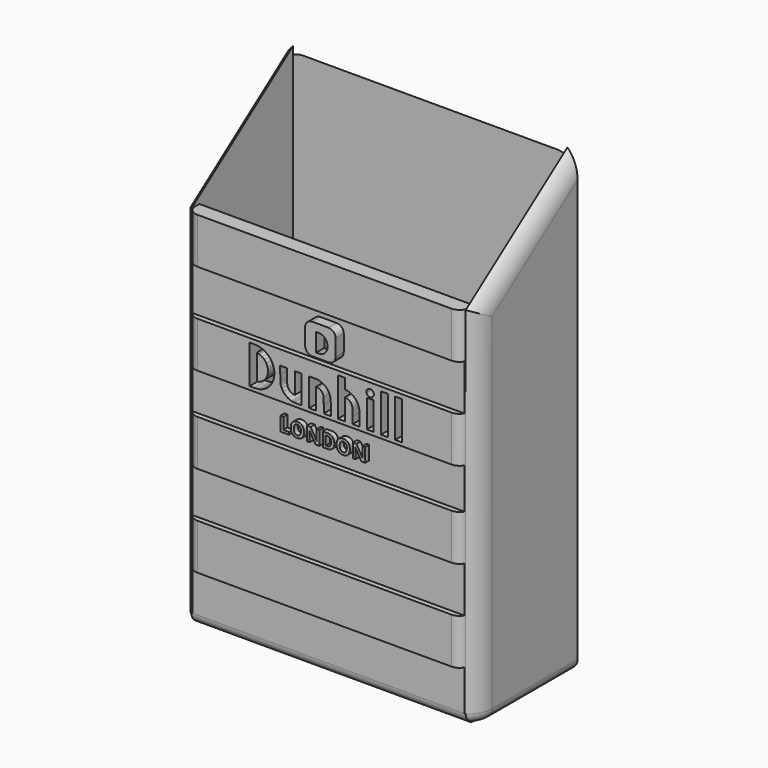
from build123d import *

# Parameters (mm, degrees)
F0_W           = 54
F0_H           = 25
F2_DEPTH       = 2
F9_DEPTH       = 2
F4_W           = 54
F4_H           = 70
F10_DEPTH      = 2
F11_DEPTH      = 2
F1_W           = 58
F1_H           = 90
F12_DEPTH      = 2
F13_T1_DEPTH   = 92
F13_2_T1_DEPTH = 92
F13_3_T1_DEPTH = 110
F14_R          = 1.99999
F14_2_R        = 1.99999
F14_3_R        = 1.99999
F15_R          = 1.99999
F16_W          = 54
F16_H          = 9
F17_DEPTH      = 1
F18_F1_R       = 2
F18_F2_R       = 1.9996
F20_DEPTH      = 3
F21_TEXT_SIZE  = 3.8399082091
F22_DEPTH      = 1
F23_W          = 6
F23_H          = 6
F24_DEPTH      = 2
F25_R          = 1.4
F27_DEPTH      = 2
F28_T1_DEPTH   = 45.8860060935
F28_2_T1_DEPTH = 45.8389282305
F28_3_T1_DEPTH = 50
F28_3_T4_ANGLE = 196.3896000127
F28_3_T6_ANGLE = 196.3896000127


# Not quite as in the source:
# - a fillet or chamfer that OpenCascade refuses, or shapes differently, is made with other operations: its cross-section is extruded or revolved along the edge and cut away or added
# - a fillet or chamfer is up to 0.001 mm smaller than in the source, because OpenCascade refuses the exact size
# - Text() gives the source's letters only with a copy of the font that has no kerning and outlines rounded to 1/6400 em; it was checked with that copy


with BuildPart() as f2:
    # F0 (on Top) → F2 (new body)
    with BuildSketch(Plane.XY):
        with Locations((23.2370707691, -12.5)):
            Rectangle(F0_W, F0_H)
    extrude(amount=-F2_DEPTH)

    # F15 (radius 2 in the source; OpenCascade refuses exactly that, so slightly less here)
    f15_edges = [f2.edges().sort_by_distance(p)[0] for p in [
        (23.237071, -25, -2),
    ]]
    fillet(f15_edges, radius=F15_R)


with BuildPart() as f9:
    # F6 (on offset) → F9 (new body)
    with BuildSketch(Plane.YZ.offset(50.2370707691)):
        Polygon((-25, 70), (-25, -2), (0, -2), (0, 88.0185291171), align=None)
    extrude(amount=F9_DEPTH)

    # F13: fillet of radius 5 on 1 edges, made by hand

    # F13_s2 → F13_t1 (cut)
    with BuildSketch(Plane.XY.offset(-12)):
        with BuildLine():
            ThreePointArc((50.2370707691, -25), (51.7092067241, -23.2360679775), (52.2370707691, -21))
            Line((52.2370707691, -21), (52.2370707691, -25))
            Line((52.2370707691, -25), (50.2370707691, -25))
        make_face()
    extrude(amount=F13_T1_DEPTH, mode=Mode.SUBTRACT)

    # F14 (radius 2 in the source; OpenCascade refuses exactly that, so slightly less here)
    f14_edges = [f9.edges().sort_by_distance(p)[0] for p in [
        (52.237071, -10.5, -2),
    ]]
    fillet(f14_edges, radius=F14_R)

    # F28: fillet of radius 5 on 1 edges, made by hand

    # F28_s2 → F28_t1 (cut)
    with BuildSketch(Plane(origin=(0, 49.8630148254, 35.9383273799), x_dir=(1, 0, 0), z_dir=(0, -0.811249133, -0.584700645))):
        with BuildLine():
            ThreePointArc((50.2370707691, 71.4049554335), (51.7092067241, 69.641023411), (52.2370707691, 67.4049554335))
            Line((52.2370707691, 67.4049554335), (52.2370707691, 71.4049554335))
            Line((52.2370707691, 71.4049554335), (50.2370707691, 71.4049554335))
        make_face()
    extrude(amount=F28_T1_DEPTH, mode=Mode.SUBTRACT)


with BuildPart() as f10:
    # F4 (on offset) → F10 (new body)
    with BuildSketch(Plane.XZ.offset(23)):
        with Locations((23.2337976322, 35)):
            Rectangle(F4_W, F4_H)
    extrude(amount=F10_DEPTH)

    # F16 (on face) → F17 (join)
    with BuildSketch(Plane.XZ.offset(25)):
        with Locations((23.2337976322, 65.5)):
            Rectangle(F16_W, F16_H)
        with Locations((23.2337976322, 47.5)):
            Rectangle(F16_W, F16_H)
        with Locations((23.2337976322, 30.5)):
            Rectangle(F16_W, F16_H)
        with Locations((23.2337976322, 12.5)):
            Rectangle(F16_W, F16_H)
    extrude(amount=F17_DEPTH)

    # F18: fillet of radius 2 on 8 edges, made by hand

    # F18_f1
    f18_f1_edges = [f10.edges().sort_by_distance(p)[0] for p in [
        (-3.7662023678, -26, 47.5),
    ]]
    fillet(f18_f1_edges, radius=F18_F1_R)

    # F18_f2 (radius 2 in the source; OpenCascade refuses exactly that, so slightly less here)
    f18_f2_edges = [f10.edges().sort_by_distance(p)[0] for p in [
        (50.2337976322, -26, 12.5),
    ]]
    fillet(f18_f2_edges, radius=F18_F2_R)

    # F19 (on face) → F20 (cut)
    with BuildSketch(Plane.XZ.offset(26)):
        with BuildLine():
            Line((8.4967808397, 51.220968125), (8.4967808397, 47.4348578924))
            Line((8.4967808397, 47.4348578924), (8.4967808397, 43.6487476599))
            Line((8.4967808397, 43.6487476599), (9.368873863, 43.668248809))
            ThreePointArc((9.3688738631, 43.6682488024), (9.7077723614, 43.6793255754), (10.0463702246, 43.6973914009))
            ThreePointArc((10.0463702223, 43.6973914371), (10.266896193, 43.7191683277), (10.4853730632, 43.7562330531))
            ThreePointArc((10.4853730706, 43.7562330175), (10.6760414895, 43.8040619553), (10.8619078322, 43.8680600487))
            ThreePointArc((10.8619078192, 43.8680600818), (11.0872012313, 43.9625459733), (11.3079983364, 44.0671086035))
            ThreePointArc((11.3079983468, 44.0671085827), (11.6452174269, 44.2584053812), (11.9611395896, 44.483137133))
            ThreePointArc((11.9611395912, 44.483137131), (12.2508833738, 44.7379466338), (12.5126747359, 45.0213979082))
            ThreePointArc((12.5126747117, 45.0213979284), (12.7444666513, 45.3313556173), (12.943023476, 45.6635851457))
            ThreePointArc((12.9430235242, 45.6635851201), (13.1084809679, 46.0179285104), (13.2376405598, 46.3870534266))
            ThreePointArc((13.2376405484, 46.3870534299), (13.2909037655, 46.5945265675), (13.3294551184, 46.8052298334))
            ThreePointArc((13.3294551154, 46.8052298339), (13.3574144288, 47.0387027013), (13.3729137893, 47.2733323517))
            ThreePointArc((13.3729137735, 47.2733323524), (13.3759300416, 47.509092507), (13.3664249519, 47.744680286))
            ThreePointArc((13.36642497, 47.7446802873), (13.3445612976, 47.9596933996), (13.3079449581, 48.1726908229))
            ThreePointArc((13.3079449225, 48.1726908155), (13.1932583708, 48.6006717625), (13.0305332816, 49.0127897571))
            ThreePointArc((13.0305333058, 49.0127897683), (12.82358236, 49.3985536561), (12.5725005259, 49.7571626126))
            ThreePointArc((12.5725005308, 49.7571626165), (12.2803608082, 50.084163496), (11.9516949748, 50.3744288275))
            ThreePointArc((11.9516949682, 50.374428819), (11.5863213494, 50.6286025823), (11.1946065561, 50.8399357408))
            ThreePointArc((11.1946065575, 50.8399357437), (10.9931829534, 50.9280602816), (10.787480949, 51.005675279))
            ThreePointArc((10.7874809466, 51.0056752723), (10.6003517758, 51.0632567232), (10.4095232186, 51.1070449848))
            ThreePointArc((10.4095232219, 51.107045002), (10.1878049733, 51.1427450964), (9.9643702521, 51.1653372164))
            ThreePointArc((9.9643702512, 51.1653372049), (9.6462722249, 51.1846554218), (9.3278341912, 51.1971760702))
            Line((9.3278341913, 51.197176073), (8.4967808397, 51.220968125))
        make_face()
        with BuildLine():
            ThreePointArc((10.3421098572, 49.8377194327), (10.3942364029, 49.821717243), (10.4461652473, 49.8050846858))
            ThreePointArc((10.4461652344, 49.8050846463), (10.7123895905, 49.6984875575), (10.9625976621, 49.5583652251))
            ThreePointArc((10.9625976924, 49.5583652719), (11.2036710915, 49.3816313865), (11.4229646443, 49.1785019016))
            ThreePointArc((11.4229646233, 49.1785018814), (11.6208645225, 48.9482688721), (11.7916159508, 48.6972398729))
            ThreePointArc((11.79161596, 48.6972398784), (11.930667684, 48.4317134841), (12.0377438832, 48.1517593172))
            ThreePointArc((12.037743906, 48.1517593244), (12.0838629347, 47.9778393221), (12.113258297, 47.8003258165))
            ThreePointArc((12.1132582866, 47.8003258153), (12.1300120701, 47.5988487204), (12.1332024594, 47.3967014215))
            ThreePointArc((12.1332024459, 47.3967014217), (12.1227781224, 47.1934925842), (12.0987956049, 46.9914348274))
            ThreePointArc((12.0987955999, 46.9914348282), (12.0628385981, 46.8111503169), (12.0107246706, 46.6348563875))
            ThreePointArc((12.0107246527, 46.6348563937), (11.8929420091, 46.3494845152), (11.7425269104, 46.0798826638))
            ThreePointArc((11.7425269194, 46.0798826581), (11.5620601339, 45.8308124438), (11.3533507512, 45.6048818663))
            ThreePointArc((11.3533507478, 45.6048818699), (11.1202369481, 45.4061489653), (10.8651243479, 45.2365778234))
            ThreePointArc((10.8651243526, 45.2365778153), (10.5925010557, 45.0992258668), (10.3053375694, 44.9956587298))
            ThreePointArc((10.3053375696, 44.9956587292), (10.1899858789, 44.9766548845), (10.0734708548, 44.986215628))
            ThreePointArc((10.0734708495, 44.9862156028), (10.0002728859, 45.0269816707), (9.9634339656, 45.1022326383))
            ThreePointArc((9.9634339712, 45.1022326392), (9.9428673797, 45.2813766604), (9.9356912782, 45.4615545409))
            ThreePointArc((9.9356912776, 45.4615545409), (9.9337995981, 46.4470459979), (9.9331693487, 47.4325390689))
            Line((9.9331693486, 47.4325390689), (9.9331693486, 49.9349330497))
            Line((9.9331693486, 49.9349330497), (10.0665482816, 49.91026714))
            ThreePointArc((10.066548282, 49.910267142), (10.10056304, 49.9033961224), (10.1343333028, 49.8954096324))
            ThreePointArc((10.1343333037, 49.895409636), (10.1837772482, 49.8825691283), (10.2330795556, 49.8691950946))
            ThreePointArc((10.233079556, 49.8691950959), (10.2876793131, 49.8537503375), (10.3421098571, 49.8377194322))
        make_face(mode=Mode.SUBTRACT)
        with BuildLine():
            Line((25.8976016332, 51.2092148555), (25.8976016332, 47.4335650607))
            Line((25.8976016332, 47.4335650607), (25.8976016332, 43.6579152659))
            Line((25.8976016332, 43.6579152659), (26.5747562159, 43.6579152659))
            Line((26.5747562159, 43.6579152659), (27.2519107987, 43.6579152659))
            Line((27.2519107987, 43.6579152659), (27.2519107987, 45.7361351428))
            Line((27.2519107987, 45.7361351428), (27.2519107987, 47.8143550196))
            Line((27.2519107987, 47.8143550196), (27.4602764348, 47.7896771674))
            ThreePointArc((27.4602764366, 47.7896771826), (27.6229020401, 47.7600920806), (27.7806130739, 47.7105986973))
            ThreePointArc((27.7806130713, 47.7105986903), (27.9373517472, 47.6403229619), (28.085370267, 47.5531667323))
            ThreePointArc((28.085370265, 47.5531667294), (28.2217245815, 47.4509514822), (28.3458536199, 47.3341934495))
            ThreePointArc((28.3458536112, 47.3341934412), (28.4492623182, 47.2101111114), (28.5355912966, 47.0735933736))
            ThreePointArc((28.5355913081, 47.0735933798), (28.6076371898, 46.9252978609), (28.6656963831, 46.7709887552))
            ThreePointArc((28.6656963911, 46.7709887578), (28.7075850332, 46.6158854669), (28.7338101803, 46.4573801645))
            ThreePointArc((28.7338101596, 46.4573801622), (28.7545565402, 46.2249601835), (28.763644156, 45.9917931317))
            ThreePointArc((28.7636441641, 45.9917931318), (28.7686951555, 45.5079692206), (28.7703786509, 45.0241218733))
            Line((28.770378651, 45.0241218733), (28.770378651, 43.6579152659))
            Line((28.770378651, 43.6579152659), (29.4475332337, 43.6579152659))
            Line((29.4475332337, 43.6579152659), (30.1246878165, 43.6579152659))
            Line((30.1246878165, 43.6579152659), (30.1243778028, 45.0224843493))
            ThreePointArc((30.1243778036, 45.0224843493), (30.1235330819, 45.2944295527), (30.1211230705, 45.566365389))
            ThreePointArc((30.1211230767, 45.5663653891), (30.1172633689, 45.8160885378), (30.1115488496, 46.0657761279))
            ThreePointArc((30.1115488419, 46.0657761277), (30.1053866555, 46.2743546576), (30.0979989786, 46.482893378))
            ThreePointArc((30.0979990012, 46.4828933789), (30.0920925158, 46.5686115086), (30.0809803833, 46.6538113023))
            ThreePointArc((30.0809803539, 46.6538112976), (29.9992595289, 47.0168027816), (29.8737606722, 47.3670757432))
            ThreePointArc((29.8737606904, 47.3670757511), (29.7073423227, 47.6960324996), (29.5008948305, 48.0014617852))
            ThreePointArc((29.5008948152, 48.0014617734), (29.2565085481, 48.2800852993), (28.9792278131, 48.525994044))
            ThreePointArc((28.9792278008, 48.5259940283), (28.6684591584, 48.7402404835), (28.3345250977, 48.9162141628))
            ThreePointArc((28.3345251138, 48.9162141984), (28.2184154982, 48.9656102913), (28.1001164396, 49.0095050471))
            ThreePointArc((28.100116427, 49.0095050105), (27.9726735504, 49.0506384212), (27.8437141442, 49.0867371167))
            ThreePointArc((27.8437141557, 49.0867371612), (27.7221838754, 49.1155868542), (27.5995860553, 49.1394968592))
            ThreePointArc((27.5995860522, 49.1394968417), (27.5030586417, 49.1521430432), (27.4058095675, 49.1566246663))
            Line((27.4058095675, 49.156624664), (27.2519107987, 49.1572312714))
            Line((27.2519107987, 49.1572312714), (27.2519107987, 50.1832230634))
            Line((27.2519107987, 50.1832230634), (27.2519107987, 51.2092148555))
            Line((27.2519107987, 51.2092148555), (26.5747562159, 51.2092148555))
            Line((26.5747562159, 51.2092148555), (25.8976016332, 51.2092148555))
        make_face()
        Polygon((34.3517739998, 51.1681751838), (34.3517739998, 47.4130452248), (34.3517739998, 43.6579152659), (35.0289285826, 43.6579152659), (35.7060831653, 43.6579152659), (35.7060831653, 47.4130452248), (35.7060831653, 51.1681751838), (35.0289285826, 51.1681751838), align=None)
        Polygon((37.1424716742, 51.1681751838), (37.1424716742, 47.4130452248), (37.1424716742, 43.6579152659), (37.819626257, 43.6579152659), (38.4967808397, 43.6579152659), (38.4967808397, 47.4130452248), (38.4967808397, 51.1681751838), (37.819626257, 51.1681751838), align=None)
        with BuildLine():
            ThreePointArc((32.1791323452, 50.8734274335), (32.0340379968, 50.8460404102), (31.896299571, 50.7928375433))
            ThreePointArc((31.8962995589, 50.7928375677), (31.7524013071, 50.6990758408), (31.6343795702, 50.5743006913))
            ThreePointArc((31.634379585, 50.5743006803), (31.5502098515, 50.4266613576), (31.5040648836, 50.2630992728))
            ThreePointArc((31.5040648713, 50.2630992747), (31.4984281146, 50.0921051918), (31.533746399, 49.9247033752))
            ThreePointArc((31.5337463815, 49.9247033692), (31.608345886, 49.7673183857), (31.7166586456, 49.6309238652))
            ThreePointArc((31.7166586768, 49.6309238964), (31.8507479036, 49.5245760291), (32.0055320329, 49.4515577919))
            ThreePointArc((32.0055320209, 49.4515577564), (32.1702777175, 49.4172739814), (32.3384419099, 49.4233834952))
            ThreePointArc((32.3384419082, 49.4233835056), (32.5000557816, 49.4695088239), (32.6459142045, 49.553006785))
            ThreePointArc((32.6459142072, 49.5530067814), (32.7700648801, 49.6701605911), (32.8640859039, 49.8126332263))
            ThreePointArc((32.8640859055, 49.8126332255), (32.9003694958, 49.8944319986), (32.9282558218, 49.9794607645))
            ThreePointArc((32.9282558337, 49.9794607613), (32.9453784748, 50.0615673922), (32.9523778003, 50.1451478511))
            ThreePointArc((32.9523778003, 50.1451478511), (32.9490635085, 50.2265235807), (32.9355120586, 50.3068314391))
            ThreePointArc((32.9355120386, 50.3068314344), (32.9117988891, 50.3860704491), (32.8787128437, 50.4618757822))
            ThreePointArc((32.8787128446, 50.4618757826), (32.7993813787, 50.5881573548), (32.6989463261, 50.6983994391))
            ThreePointArc((32.6989463218, 50.6983994344), (32.5855016264, 50.7825875652), (32.4570587006, 50.8414072481))
            ThreePointArc((32.4570587041, 50.8414072585), (32.319784733, 50.8720792133), (32.179132345, 50.8734274359))
        make_face()
        with BuildLine():
            Line((14.5241674334, 49.1572312714), (14.5396058192, 47.649023337))
            ThreePointArc((14.5396058039, 47.6490233369), (14.5467193462, 47.1057908162), (14.5569389503, 46.5626078511))
            ThreePointArc((14.5569389723, 46.5626078515), (14.5682483481, 46.3277414503), (14.5919581248, 46.0938013407))
            ThreePointArc((14.591958115, 46.0938013394), (14.6227813362, 45.9232944126), (14.6709369932, 45.7568500803))
            ThreePointArc((14.6709369781, 45.7568500751), (14.7464050066, 45.5567226203), (14.8327948173, 45.3610616327))
            ThreePointArc((14.8327948066, 45.3610616276), (14.9765414947, 45.0939940481), (15.1464320066, 44.8427463291))
            ThreePointArc((15.1464320149, 44.8427463353), (15.3378461137, 44.6146663753), (15.5524214036, 44.4082268678))
            ThreePointArc((15.5524214239, 44.4082268912), (15.7931668258, 44.2209742962), (16.0519744034, 44.0596035411))
            ThreePointArc((16.0519743908, 44.0596035182), (16.3418650995, 43.9150619759), (16.6431556653, 43.7960961178))
            ThreePointArc((16.643155674, 43.796096143), (16.7521732863, 43.7610037313), (16.862592786, 43.7306088099))
            ThreePointArc((16.8625927853, 43.7306088074), (16.95719232, 43.7102578507), (17.0529921133, 43.6966331311))
            ThreePointArc((17.052992113, 43.6966331283), (17.182524932, 43.6853873594), (17.3123959973, 43.679164428))
            ThreePointArc((17.3123959963, 43.6791643911), (17.5882244819, 43.6719989595), (17.8640859008, 43.6662392338))
            Line((17.8640859013, 43.6662392604), (18.7566987604, 43.6498773999))
            Line((18.7566987604, 43.6498773999), (18.7566987604, 46.4035543357))
            Line((18.7566987604, 46.4035543357), (18.7566987604, 49.1572312714))
            Line((18.7566987604, 49.1572312714), (18.0795441776, 49.1572312714))
            Line((18.0795441776, 49.1572312714), (17.4023895949, 49.1572312714))
            Line((17.4023895949, 49.1572312714), (17.4023895949, 47.0811205463))
            Line((17.4023895949, 47.0811205463), (17.4023895949, 45.0050098213))
            Line((17.4023895949, 45.0050098213), (17.2279709902, 45.0340384943))
            ThreePointArc((17.22797099, 45.0340384932), (17.1864201049, 45.0417336558), (17.1451768588, 45.0509361683))
            ThreePointArc((17.145176862, 45.0509361814), (17.091714273, 45.0643642451), (17.038483114, 45.0786822413))
            ThreePointArc((17.0384831181, 45.0786822558), (16.9826073956, 45.0947100997), (16.9270036524, 45.1116574263))
            ThreePointArc((16.9270036391, 45.1116573839), (16.8772295139, 45.1278964082), (16.8278341858, 45.145253568))
            ThreePointArc((16.8278341929, 45.1452535875), (16.705645414, 45.1996183167), (16.5921582152, 45.2703733671))
            ThreePointArc((16.5921582341, 45.2703733932), (16.4667498542, 45.3693126192), (16.3498733129, 45.478198368))
            ThreePointArc((16.3498733067, 45.4781983619), (16.2401345989, 45.5985830867), (16.1405164838, 45.7274679078))
            ThreePointArc((16.1405164615, 45.7274678919), (16.0646729637, 45.8489941712), (16.0037899213, 45.9786634731))
            ThreePointArc((16.0037899231, 45.9786634738), (15.9709237931, 46.0730990143), (15.9465946961, 46.1700853477))
            ThreePointArc((15.9465946649, 46.1700853413), (15.9283888077, 46.277981146), (15.9175671406, 46.3868657152))
            ThreePointArc((15.917567196, 46.3868657188), (15.9081505372, 46.5671045351), (15.9033557332, 46.7475254714))
            ThreePointArc((15.9033556986, 46.7475254709), (15.8973680354, 47.2187884673), (15.8923709791, 47.6900630086))
            Line((15.8923709902, 47.6900630087), (15.8783553678, 49.1572312714))
            Line((15.8783553678, 49.1572312714), (15.2012614006, 49.1572312714))
            Line((15.2012614006, 49.1572312714), (14.5241674334, 49.1572312714))
        make_face()
        with BuildLine():
            Line((20.234126941, 49.1572312714), (20.234126941, 46.4075732686))
            Line((20.234126941, 46.4075732686), (20.234126941, 43.6579152659))
            Line((20.234126941, 43.6579152659), (20.9112815237, 43.6579152659))
            Line((20.9112815237, 43.6579152659), (21.5884361065, 43.6579152659))
            Line((21.5884361065, 43.6579152659), (21.5884361065, 45.7304186859))
            Line((21.5884361065, 45.7304186859), (21.5884361065, 47.8029221058))
            Line((21.5884361065, 47.8029221058), (21.7072322077, 47.8029221058))
            ThreePointArc((21.7072322077, 47.8029221058), (21.7388715452, 47.8015985367), (21.7702897864, 47.7976370168))
            ThreePointArc((21.7702897858, 47.7976370136), (21.8202969528, 47.7886311323), (21.8700950251, 47.7785328826))
            ThreePointArc((21.8700950252, 47.7785328831), (21.9268009471, 47.7657297455), (21.9832103329, 47.7516775887))
            ThreePointArc((21.9832103366, 47.7516776032), (22.0392009393, 47.7364057299), (22.0948388186, 47.7198950037))
            ThreePointArc((22.0948388063, 47.7198949639), (22.2266138218, 47.670790851), (22.3519319459, 47.6069846099))
            ThreePointArc((22.3519319597, 47.6069846335), (22.4741158004, 47.5270829932), (22.5875148594, 47.4351383551))
            ThreePointArc((22.5875148652, 47.4351383615), (22.6946268006, 47.3288223536), (22.7907531671, 47.2124789745))
            ThreePointArc((22.790753173, 47.2124789789), (22.8774322212, 47.0845045132), (22.9520156122, 46.9491234249))
            Line((22.9520156003, 46.9491234191), (23.0863841229, 46.6763073179))
            Line((23.0863841229, 46.6763073179), (23.0985330969, 45.1671112714))
            Line((23.0985330969, 45.1671112714), (23.1106820709, 43.6579152659))
            Line((23.1106820709, 43.6579152659), (23.8107081448, 43.6579152659))
            Line((23.8107081448, 43.6579152659), (24.5107342187, 43.6579152659))
            Line((24.5107342187, 43.6579152659), (24.4920899369, 45.1250835285))
            ThreePointArc((24.4920899461, 45.1250835287), (24.4859677505, 45.5591087561), (24.4786329147, 45.993115184))
            ThreePointArc((24.4786329384, 45.9931151844), (24.4727039553, 46.2012171195), (24.462536358, 46.4091550626))
            ThreePointArc((24.4625363094, 46.4091550597), (24.4517072238, 46.5436971447), (24.4351662966, 46.6776569874))
            ThreePointArc((24.4351663012, 46.677656988), (24.4143661357, 46.7956646918), (24.3864470798, 46.9121936211))
            ThreePointArc((24.3864470891, 46.9121936236), (24.2563150281, 47.2951526976), (24.0797700986, 47.6590536366))
            ThreePointArc((24.0797701199, 47.6590536486), (23.8635396326, 47.9884802192), (23.6051821381, 48.2860182741))
            ThreePointArc((23.6051821309, 48.286018267), (23.3095967134, 48.5460553732), (22.9818479568, 48.7641626592))
            ThreePointArc((22.981847965, 48.7641626735), (22.6198876075, 48.9424100474), (22.2385495739, 49.0742005282))
            ThreePointArc((22.2385495665, 49.0742005018), (22.1411932831, 49.0985285658), (22.042724957, 49.1178699561))
            ThreePointArc((22.0427249532, 49.1178699335), (21.9416357096, 49.1325652238), (21.8399551198, 49.1423654476))
            ThreePointArc((21.8399551221, 49.1423654792), (21.7014746782, 49.1502961069), (21.562820621, 49.1541406635))
            ThreePointArc((21.5628206209, 49.1541406557), (21.3246778158, 49.156458515), (21.0865249847, 49.1572312713))
            Line((21.0865249847, 49.1572312714), (20.234126941, 49.1572312714))
        make_face()
        Polygon((31.5610763254, 49.1572312714), (31.5610763254, 46.4075732686), (31.5610763254, 43.6579152659), (32.2382309081, 43.6579152659), (32.9153854909, 43.6579152659), (32.9153854909, 46.4075732686), (32.9153854909, 49.1572312714), (32.2382309081, 49.1572312714), align=None)
    extrude(amount=-F20_DEPTH, mode=Mode.SUBTRACT)

    # F21 (on face) → F22 (join)
    with BuildSketch(Plane.XZ.offset(25)):
        with Locations((14.2162481109, 37.7536155283)):
            Text('LONDON', F21_TEXT_SIZE, font='Open Sans', font_style=FontStyle.BOLD, text_align=(TextAlign.LEFT, TextAlign.BOTTOM))
    extrude(amount=F22_DEPTH)

    # F23 (on face) → F24 (join)
    with BuildSketch(Plane.XZ.offset(25)):
        with Locations((23.2337976322, 56.5)):
            Rectangle(F23_W, F23_H)
    extrude(amount=F24_DEPTH)

    # F25
    f25_edges = [f10.edges().sort_by_distance(p)[0] for p in [
        (20.233798, -26, 59.5),
        (26.233798, -26, 59.5),
        (20.233798, -26, 53.5),
        (26.233798, -26, 53.5),
    ]]
    fillet(f25_edges, radius=F25_R)

    # F26 (on face) → F27 (cut)
    with BuildSketch(Plane.XZ.offset(27)):
        with BuildLine():
            Line((22.4137958139, 54.3826669455), (22.8759404272, 54.3826669455))
            ThreePointArc((22.8759404272, 54.3826669455), (24.6678479016, 56.1745744199), (22.8759404272, 57.9664818943))
            Line((22.8759404272, 57.9664818943), (22.4137958139, 57.9664818943))
            Line((22.4137958139, 57.9664818943), (22.4137958139, 54.3826669455))
        make_face()
    extrude(amount=-F27_DEPTH, mode=Mode.SUBTRACT)


with BuildPart() as f11:
    # F8 (on offset) → F11 (new body)
    with BuildSketch(Plane(origin=(-3.7629292309, 0, 0), x_dir=(0, -1, 0), z_dir=(-1, 0, 0))):
        Polygon((0, 88.0000001378), (0, -2), (24.9567795545, -2), (24.9567795545, 70), align=None)
    extrude(amount=F11_DEPTH)

    # F13#2: fillet of radius 5 on 1 edges, made by hand

    # F13_2_s2 → F13_2_t1 (cut)
    with BuildSketch(Plane.XY.offset(-12)):
        with BuildLine():
            ThreePointArc((-3.7629292309, -24.9567795545), (-5.2350651859, -23.192847532), (-5.7629292309, -20.9567795545))
            Line((-5.7629292309, -20.9567795545), (-5.7629292309, -24.9567795545))
            Line((-5.7629292309, -24.9567795545), (-3.7629292309, -24.9567795545))
        make_face()
    extrude(amount=F13_2_T1_DEPTH, mode=Mode.SUBTRACT)

    # F14#2 (radius 2 in the source; OpenCascade refuses exactly that, so slightly less here)
    f14_2_edges = [f11.edges().sort_by_distance(p)[0] for p in [
        (-5.762929, -10.47839, -2),
    ]]
    fillet(f14_2_edges, radius=F14_2_R)

    # F28#2: fillet of radius 5 on 1 edges, made by hand

    # F28_2_s2 → F28_2_t1 (cut)
    with BuildSketch(Plane(origin=(0, 12.6836613191, 9.1480515342), x_dir=(1, 0, 0), z_dir=(0, 0.8110545208, 0.584970567))):
        with BuildLine():
            ThreePointArc((-5.7629292309, -67.3727979439), (-5.2350651859, -69.6088659214), (-3.7629292309, -71.3727979439))
            Line((-3.7629292309, -71.3727979439), (-5.7629292309, -71.3727979439))
            Line((-5.7629292309, -71.3727979439), (-5.7629292309, -67.3727979439))
        make_face()
    extrude(amount=F28_2_T1_DEPTH, mode=Mode.SUBTRACT)


with BuildPart() as f12:
    # F1 (on Front) → F12 (new body)
    with BuildSketch(Plane.XZ):
        with Locations((23.2365219835, 43.0000001378)):
            Rectangle(F1_W, F1_H)
    extrude(amount=-F12_DEPTH)

    # F13#3: fillet of radius 5 on 2 edges, made by hand

    # F13_3_s2 → F13_3_t1 (cut)
    with BuildSketch(Plane.XY.offset(-11.9999998622)):
        with BuildLine():
            ThreePointArc((-5.7634780165, 0), (-3.999545994, 1.472135955), (-1.7634780165, 2))
            Line((-1.7634780165, 2), (-5.7634780165, 2))
            Line((-5.7634780165, 2), (-5.7634780165, 0))
        make_face()
        with BuildLine():
            ThreePointArc((52.2365219835, 0), (50.472589961, 1.472135955), (48.2365219835, 2))
            Line((48.2365219835, 2), (52.2365219835, 2))
            Line((52.2365219835, 2), (52.2365219835, 0))
        make_face()
    extrude(amount=F13_3_T1_DEPTH, mode=Mode.SUBTRACT)

    # F14#3 (radius 2 in the source; OpenCascade refuses exactly that, so slightly less here)
    f14_3_edges = [f12.edges().sort_by_distance(p)[0] for p in [
        (23.236522, 2, -2),
    ]]
    fillet(f14_3_edges, radius=F14_3_R)

    # F28#3: fillet of radius 5 on 1 edges, made by hand

    # F28_3_s2 → F28_3_t1 (cut)
    with BuildSketch(Plane.YZ.offset(-1.7634780165)):
        with BuildLine():
            ThreePointArc((-3, 88.0000001378), (0.5355339059, 86.5355340438), (2, 83.0000001378))
            Line((2, 83.0000001378), (2, 88.0000001378))
            Line((2, 88.0000001378), (-3, 88.0000001378))
        make_face()
    extrude(amount=F28_3_T1_DEPTH, mode=Mode.SUBTRACT)

    # F28_3_s3 → F28_3_t4 (revolve, cut)
    with BuildSketch(Plane.YZ.offset(48.2365219835)):
        with BuildLine():
            ThreePointArc((2, 83.0000001378), (0.5355339059, 86.5355340438), (-3, 88.0000001378))
            Line((-3, 88.0000001378), (2, 88.0000001378))
            Line((2, 88.0000001378), (2, 83.0000001378))
        make_face()
    revolve(axis=Axis((48.2365219835, -3, 88.0000001378), (0, 0, -1)), revolution_arc=F28_3_T4_ANGLE, mode=Mode.SUBTRACT)

    # F28_3_s5 → F28_3_t6 (revolve, cut)
    with BuildSketch(Plane(origin=(-2.4351772594, -0.7162313616, 0), x_dir=(0, 0, 1), z_dir=(0.9593652077, 0.2821673233, 0))):
        with BuildLine():
            ThreePointArc((88.0000001378, 2.3804997515), (86.5355340438, 5.9160336574), (83.0000001378, 7.3804997515))
            Line((83.0000001378, 7.3804997515), (88.0000001378, 7.3804997515))
            Line((88.0000001378, 7.3804997515), (88.0000001378, 2.3804997515))
        make_face()
    revolve(axis=Axis((-1.7634780165, -3, 88.0000001378), (0, 0, -1)), revolution_arc=F28_3_T6_ANGLE, mode=Mode.SUBTRACT)


solid = Compound([f2.part, f9.part, f10.part, f11.part, f12.part])
